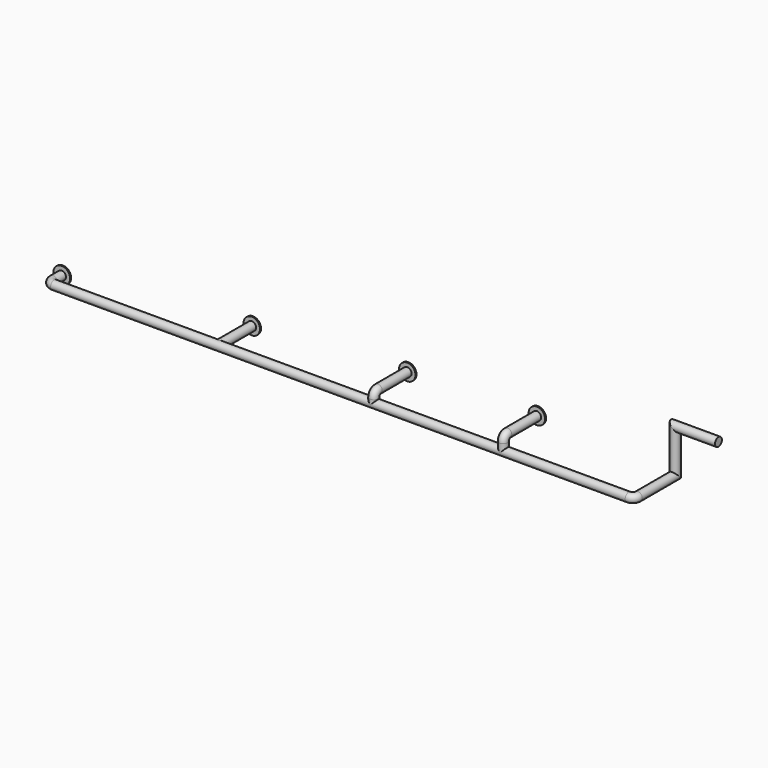
from build123d import *

# Parameters (mm, degrees)
F2_R      = 50
F2_R_2    = 97.5
F9_DEPTH  = 15
F14_R     = 50
F14_R_2   = 95
F18_DEPTH = 15


# Not quite as in the source:
# - a feature names something its author has since deleted; it is built from what else it names


with BuildPart() as f8:
    # F8: sweep along a path in F0, F5, F7
    with BuildLine(Plane.XY) as f8_path:
        Line((0, 200), (0, 60))
        ThreePointArc((0, 60), (17.5735931288, 17.5735931288), (60, 0))
        Line((60, 0), (6710, 0))
        ThreePointArc((6710, 0), (6752.4264068712, 17.5735931288), (6770, 60))
        Line((6770, 60), (6770, 540))
        Line((6770, 540), (6770, 600))
    with BuildLine(Plane.YZ.offset(6770)) as f8_path_2:
        Line((600, 0), (600, 500))
    with BuildLine(Plane.XZ.offset(-600)) as f8_path_3:
        Line((6770, 500), (7270, 500))
    # F2 (on offset) → F8 (sweep)
    with BuildSketch(Plane.XZ.offset(-200)):
        Circle(F2_R)
    sweep(path=f8_path.line + f8_path_2.line + f8_path_3.line, transition=Transition.RIGHT)

    # F2 (on offset) → F9 (join)
    with BuildSketch(Plane.XZ.offset(-200)):
        Circle(F2_R_2)
        Circle(F2_R, mode=Mode.SUBTRACT)
        Circle(F2_R)
    extrude(amount=F9_DEPTH)

    # F15: sweep along a path in F0
    with BuildLine(Plane.XY) as f15_path:
        Line((1960.38051, 0), (1960.38051, 500))
    # F14 (on offset) → F15 (sweep)
    with BuildSketch(Plane.XZ.offset(-500)):
        with Locations((1960.38051, 0)):
            Circle(F14_R)
    sweep(path=f15_path.line)

    # F16: sweep along a path in F11
    with BuildLine(Plane.YZ.offset(3760)) as f16_path:
        Line((500, 117), (60, 117))
        ThreePointArc((60, 117), (17.5735931288, 99.4264068712), (0, 57))
        Line((0, 57), (0, 0))
    # F14 (on offset) → F16 (sweep)
    with BuildSketch(Plane.XZ.offset(-500)):
        with Locations((3760, 117)):
            Circle(F14_R)
    sweep(path=f16_path.line)

    # F17: sweep along a path in F13
    with BuildLine(Plane.YZ.offset(5260)) as f17_path:
        Line((500, 157), (60, 157))
        ThreePointArc((60, 157), (17.5735931288, 139.4264068712), (0, 97))
        Line((0, 97), (0, 0))
    # F14 (on offset) → F17 (sweep)
    with BuildSketch(Plane.XZ.offset(-500)):
        with Locations((5260, 157)):
            Circle(F14_R)
    sweep(path=f17_path.line)

    # F14 (on offset) → F18 (join)
    with BuildSketch(Plane.XZ.offset(-500)):
        with Locations((1960.38051, 0)):
            Circle(F14_R_2)
        with Locations((1960.38051, 0)):
            Circle(F14_R, mode=Mode.SUBTRACT)
        with Locations((3760, 117)):
            Circle(F14_R_2)
        with Locations((3760, 117)):
            Circle(F14_R, mode=Mode.SUBTRACT)
        with Locations((5260, 157)):
            Circle(F14_R_2)
        with Locations((5260, 157)):
            Circle(F14_R, mode=Mode.SUBTRACT)
        with Locations((1960.38051, 0)):
            Circle(F14_R)
        with Locations((3760, 117)):
            Circle(F14_R)
        with Locations((5260, 157)):
            Circle(F14_R)
    extrude(amount=F18_DEPTH)


solid = f8.part
